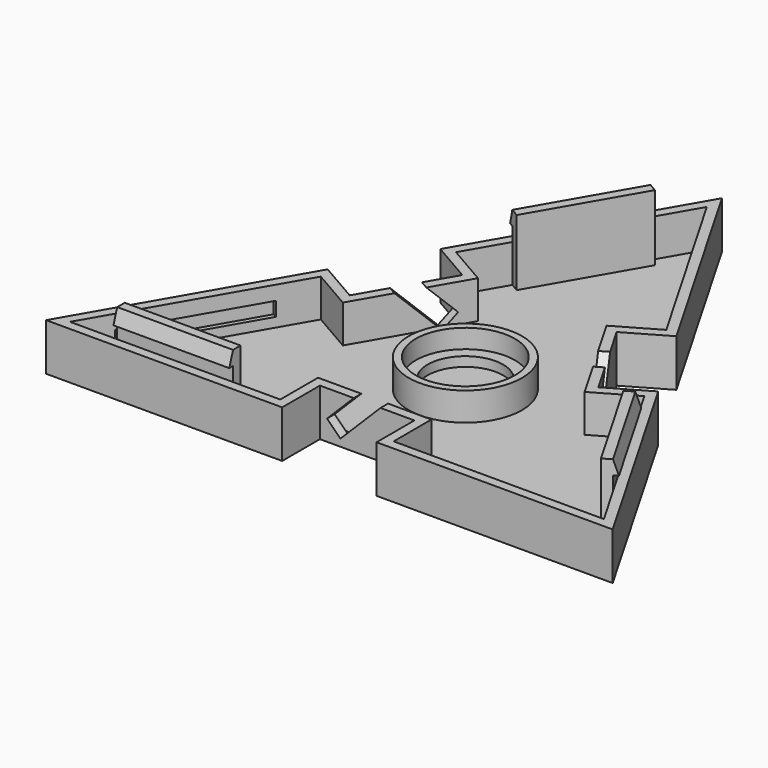
from build123d import *

# Parameters (mm, degrees)
F1_DEPTH     = 10
F2_W         = 10
F2_H         = 10
F3_DEPTH     = 5
F4_W         = 10
F4_H         = 10
F5_DEPTH     = 5
F6_W         = 10
F6_H         = 10
F7_DEPTH     = 5
F9_DEPTH     = 9
F10_DEPTH    = 5
F11_W        = 12.2679491924
F11_H        = 4
F11_H_2      = 3
F12_DEPTH    = 1
F13_W        = 12.2679491924
F13_H        = 4
F13_H_2      = 3
F14_DEPTH    = 1
F15_W        = 12.2679491924
F15_H        = 4
F15_H_2      = 3
F16_DEPTH    = 1
F17_W        = 12.2679491924
F17_H        = 1.5
F18_DEPTH    = 0.5
F19_T1_DEPTH = 20.0531322244
F20_W        = 12.2679491924
F20_H        = 1.5
F21_DEPTH    = 0.5
F22_T1_DEPTH = 20.0531322244
F23_W        = 12.2679491924
F23_H        = 1.5
F24_DEPTH    = 0.5
F25_T1_DEPTH = 20.0531322244
F26_W        = 14.2679491924
F26_H        = 1.5
F27_DEPTH    = 0.5
F28_W        = 14.2679491924
F28_H        = 1.5
F29_DEPTH    = 0.5
F30_W        = 14.2679491924
F30_H        = 1.5
F31_DEPTH    = 0.5
F32_R        = 6
F33_DEPTH    = 4
F34_R        = 5.25
F35_DEPTH    = 3
F36_R        = 4
F37_DEPTH    = 1
F39_DEPTH    = 1
F41_DEPTH    = 1
F43_DEPTH    = 1
F44_DEPTH    = 1


# Not quite as in the source:
# - a fillet or chamfer that OpenCascade refuses, or shapes differently, is made with other operations: its cross-section is extruded or revolved along the edge and cut away or added


with BuildPart() as f1:
    # F0 (on Top) → F1 (new body)
    with BuildSketch(Plane.XY):
        Polygon((30, 51.9615242271), (0, 0), (60, 0), align=None)
    extrude(amount=F1_DEPTH)

    # F2 (on face) → F3 (cut)
    with BuildSketch(Plane.XZ):
        with Locations((30, 5)):
            Rectangle(F2_W, F2_H)
    extrude(amount=-F3_DEPTH, mode=Mode.SUBTRACT)

    # F4 (on face) → F5 (cut)
    with BuildSketch(Plane(origin=(0, 0, 0), x_dir=(-0.5, -0.8660254038, 0), z_dir=(-0.8660254038, 0.5, 0))):
        with Locations((-30, 5)):
            Rectangle(F4_W, F4_H)
    extrude(amount=-F5_DEPTH, mode=Mode.SUBTRACT)

    # F6 (on face) → F7 (cut)
    with BuildSketch(Plane(origin=(45, 25.9807621135, 0), x_dir=(-0.5, 0.8660254038, 0), z_dir=(0.8660254038, 0.5, 0))):
        with Locations((0, 5)):
            Rectangle(F6_W, F6_H)
    extrude(amount=-F7_DEPTH, mode=Mode.SUBTRACT)

    # F8 (on face) → F9 (cut)
    with BuildSketch(Plane.XY.offset(10)):
        Polygon((18.8660254038, 30.6769145362), (23.1961524227, 28.1769145362), (17.1961524227, 17.7846096908), (12.8660254038, 20.2846096908), (1.7320508076, 1), (24, 1), (24, 6), (36, 6), (36, 1), (58.2679491924, 1), (47.1339745962, 20.2846096908), (42.8038475773, 17.7846096908), (36.8038475773, 28.1769145362), (41.1339745962, 30.6769145362), (30, 49.9615242271), align=None)
    extrude(amount=-F9_DEPTH, mode=Mode.SUBTRACT)

    # F10 (cut): a face of the model
    f10_faces = [f1.faces().sort_by_distance(p)[0] for p in [
        (35.7937253933, 2.5, 10),
    ]]
    extrude(f10_faces, amount=-F10_DEPTH, mode=Mode.SUBTRACT)

    # F11 (on face) → F12 (join)
    with BuildSketch(Plane(origin=(0.8660254038, -0.5, 0), x_dir=(0.5, 0.8660254038, 0), z_dir=(0.8660254038, -0.5, 0))):
        with Locations((47.1339745962, 3)):
            Rectangle(F11_W, F11_H)
        with Locations((47.1339745962, 6.5)):
            Rectangle(F11_W, F11_H_2)
    extrude(amount=F12_DEPTH)

    # F13 (on face) → F14 (join)
    with BuildSketch(Plane(origin=(0, 1, 0), x_dir=(-1, 0, 0), z_dir=(0, 1, 0))):
        with Locations((-12.8660254038, 3)):
            Rectangle(F13_W, F13_H)
        with Locations((-12.8660254038, 6.5)):
            Rectangle(F13_W, F13_H_2)
    extrude(amount=F14_DEPTH)

    # F15 (on face) → F16 (join)
    with BuildSketch(Plane(origin=(44.1339745962, 25.4807621135, 0), x_dir=(0.5, -0.8660254038, 0), z_dir=(-0.8660254038, -0.5, 0))):
        with Locations((17.1339745962, 3)):
            Rectangle(F15_W, F15_H)
        with Locations((17.1339745962, 6.5)):
            Rectangle(F15_W, F15_H_2)
    extrude(amount=F16_DEPTH)

    # F17 (on face) → F18 (join)
    with BuildSketch(Plane.XZ.offset(-1)):
        with Locations((12.8660254038, 7.25)):
            Rectangle(F17_W, F17_H)
    extrude(amount=F18_DEPTH)

    # F19: chamfer of 0.5 x 1.5 on 1 edges, made by hand

    # F19_s2 → F19_t1 (cut)
    with BuildSketch(Plane.YZ.offset(2.8394592916)):
        Polygon((0.5, 6.5), (1, 8), (0.5, 8), align=None)
    extrude(amount=F19_T1_DEPTH, mode=Mode.SUBTRACT)

    # F20 (on face) → F21 (join)
    with BuildSketch(Plane(origin=(44.1339745962, 25.4807621135, 0), x_dir=(-0.5, 0.8660254038, 0), z_dir=(0.8660254038, 0.5, 0))):
        with Locations((-17.1339745962, 7.25)):
            Rectangle(F20_W, F20_H)
    extrude(amount=F21_DEPTH)

    # F22: chamfer of 0.5 x 1.5 on 1 edges, made by hand

    # F22_s2 → F22_t1 (cut)
    with BuildSketch(Plane(origin=(3.553704242, -6.1551963022, 0), x_dir=(0, 0, 1), z_dir=(0.5, -0.8660254038, 0))):
        Polygon((6.5, -51.4615242271), (8, -50.9615242271), (8, -51.4615242271), align=None)
    extrude(amount=F22_T1_DEPTH, mode=Mode.SUBTRACT)

    # F23 (on face) → F24 (join)
    with BuildSketch(Plane(origin=(0.8660254038, -0.5, 0), x_dir=(-0.5, -0.8660254038, 0), z_dir=(-0.8660254038, 0.5, 0))):
        with Locations((-47.1339745962, 7.25)):
            Rectangle(F23_W, F23_H)
    extrude(amount=F24_DEPTH)

    # F25: chamfer of 0.5 x 1.5 on 1 edges, made by hand

    # F25_s2 → F25_t1 (cut)
    with BuildSketch(Plane(origin=(18.553704242, 32.1359584158, 0), x_dir=(0, 0, 1), z_dir=(0.5, 0.8660254038, 0))):
        Polygon((6.5, 0.5), (8, 1), (8, 0.5), align=None)
    extrude(amount=F25_T1_DEPTH, mode=Mode.SUBTRACT)

    # F26 (on face) → F27 (cut)
    with BuildSketch(Plane(origin=(44.1339745962, 25.4807621135, 0), x_dir=(0.5, -0.8660254038, 0), z_dir=(-0.8660254038, -0.5, 0))):
        with Locations((-17.1339745962, 2.75)):
            Rectangle(F26_W, F26_H)
    extrude(amount=-F27_DEPTH, mode=Mode.SUBTRACT)

    # F28 (on face) → F29 (cut)
    with BuildSketch(Plane(origin=(0, 1, 0), x_dir=(-1, 0, 0), z_dir=(0, 1, 0))):
        with Locations((-47.1339745962, 2.75)):
            Rectangle(F28_W, F28_H)
    extrude(amount=-F29_DEPTH, mode=Mode.SUBTRACT)

    # F30 (on face) → F31 (cut)
    with BuildSketch(Plane(origin=(0.8660254038, -0.5, 0), x_dir=(0.5, 0.8660254038, 0), z_dir=(0.8660254038, -0.5, 0))):
        with Locations((12.8660254038, 2.75)):
            Rectangle(F30_W, F30_H)
    extrude(amount=-F31_DEPTH, mode=Mode.SUBTRACT)

    # F32 (on face) → F33 (join)
    with BuildSketch(Plane.XY.offset(1)):
        with Locations((30, 18)):
            Circle(F32_R)
    extrude(amount=F33_DEPTH)

    # F34 (on face) → F35 (cut)
    with BuildSketch(Plane.XY.offset(5)):
        with Locations((30, 18)):
            Circle(F34_R)
    extrude(amount=-F35_DEPTH, mode=Mode.SUBTRACT)

    # F36 (on face) → F37 (cut)
    with BuildSketch(Plane.XY.offset(2)):
        with Locations((30, 18)):
            Circle(F36_R)
    extrude(amount=-F37_DEPTH, mode=Mode.SUBTRACT)

    # F38 (on face) → F39 (cut)
    with BuildSketch(Plane.XZ.offset(-5)):
        Polygon((25.7573593129, 2.1715728753), (27.1715728753, 0.7573593129), (31.4142135624, 5), (28.5857864376, 5), align=None)
    extrude(amount=-F39_DEPTH, mode=Mode.SUBTRACT)

    # F40 (on face) → F41 (cut)
    with BuildSketch(Plane(origin=(40.6698729811, 23.4807621135, 0), x_dir=(-0.5, 0.8660254038, 0), z_dir=(0.8660254038, 0.5, 0))):
        Polygon((-4.2426406871, 2.1715728753), (-2.8284271247, 0.7573593129), (1.4142135624, 5), (-1.4142135624, 5), align=None)
    extrude(amount=-F41_DEPTH, mode=Mode.SUBTRACT)

    # F42 (on face) → F43 (cut)
    with BuildSketch(Plane(origin=(4.3301270189, -2.5, 0), x_dir=(-0.5, -0.8660254038, 0), z_dir=(-0.8660254038, 0.5, 0))):
        Polygon((-34.2426406871, 2.1715728753), (-32.8284271247, 0.7573593129), (-28.5857864376, 5), (-31.4142135624, 5), align=None)
    extrude(amount=-F43_DEPTH, mode=Mode.SUBTRACT)

    # F44 (cut): a face of the model
    f44_faces = [f1.faces().sort_by_distance(p)[0] for p in [
        (24.1697056275, 18, 5),
    ]]
    extrude(f44_faces, amount=-F44_DEPTH, mode=Mode.SUBTRACT)


solid = f1.part
